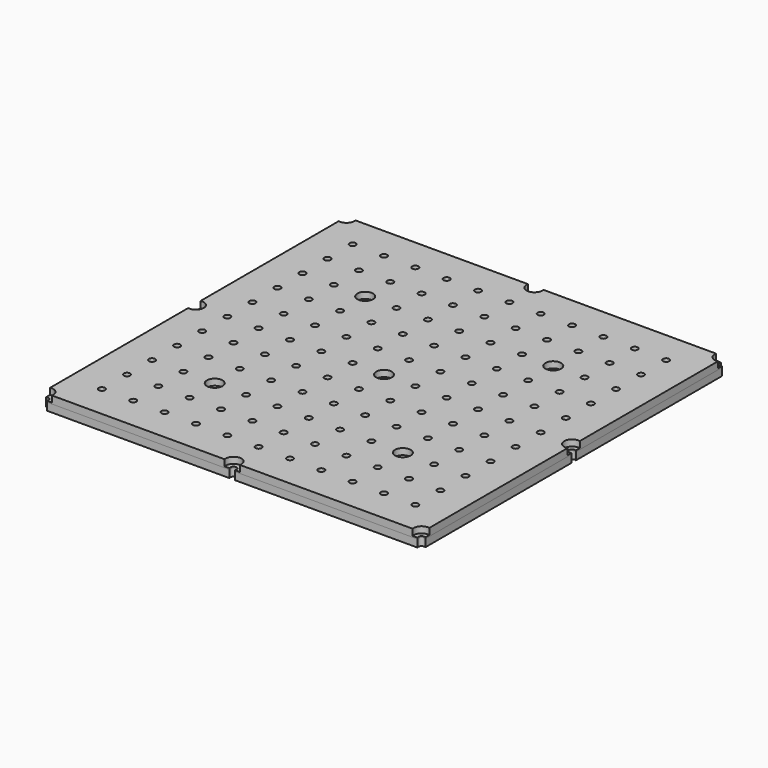
from build123d import *

# Parameters (mm, degrees)
F0_R     = 5
F1_DEPTH = 12
F2_R     = 5
F2_R_2   = 12.5
F3_DEPTH = 12
F4_R     = 5
F5_DEPTH = 2


with BuildPart() as f1:
    # F0 (on Top) → F1 (new body)
    with BuildSketch(Plane.XY):
        with BuildLine():
            ThreePointArc((302.5, 295.6698729811), (296.4644660941, 296.4644660941), (295.6698729811, 302.5))
            Line((295.6698729811, 302.5), (4.3301270189, 302.5))
            ThreePointArc((4.3301270189, 302.5), (0, 295), (-4.3301270189, 302.5))
            Line((-4.3301270189, 302.5), (-295.6698729811, 302.5))
            ThreePointArc((-295.6698729811, 302.5), (-296.4644660941, 296.4644660941), (-302.5, 295.6698729811))
            Line((-302.5, 295.6698729811), (-302.5, 4.3301270189))
            ThreePointArc((-302.5, 4.3301270189), (-295, 0), (-302.5, -4.3301270189))
            Line((-302.5, -4.3301270189), (-302.5, -295.6698729811))
            ThreePointArc((-302.5, -295.6698729811), (-296.4644660941, -296.4644660941), (-295.6698729811, -302.5))
            Line((-295.6698729811, -302.5), (-4.3301270189, -302.5))
            ThreePointArc((-4.3301270189, -302.5), (0, -295), (4.3301270189, -302.5))
            Line((4.3301270189, -302.5), (295.6698729811, -302.5))
            ThreePointArc((295.6698729811, -302.5), (296.4644660941, -296.4644660941), (302.5, -295.6698729811))
            Line((302.5, -295.6698729811), (302.5, -4.3301270189))
            ThreePointArc((302.5, -4.3301270189), (295, 0), (302.5, 4.3301270189))
            Line((302.5, 4.3301270189), (302.5, 295.6698729811))
        make_face()
        with Locations((-250, -250)):
            Circle(F0_R, mode=Mode.SUBTRACT)
        with Locations((-200, -250)):
            Circle(F0_R, mode=Mode.SUBTRACT)
        with Locations((-250, -200)):
            Circle(F0_R, mode=Mode.SUBTRACT)
        with Locations((-200, -200)):
            Circle(F0_R, mode=Mode.SUBTRACT)
        with Locations((-150, -250)):
            Circle(F0_R, mode=Mode.SUBTRACT)
        with Locations((-100, -250)):
            Circle(F0_R, mode=Mode.SUBTRACT)
        with Locations((-50, -250)):
            Circle(F0_R, mode=Mode.SUBTRACT)
        with Locations((-150, -200)):
            Circle(F0_R, mode=Mode.SUBTRACT)
        with Locations((-100, -200)):
            Circle(F0_R, mode=Mode.SUBTRACT)
        with Locations((-50, -200)):
            Circle(F0_R, mode=Mode.SUBTRACT)
        with Locations((-250, -150)):
            Circle(F0_R, mode=Mode.SUBTRACT)
        with Locations((-250, -100)):
            Circle(F0_R, mode=Mode.SUBTRACT)
        with Locations((-200, -150)):
            Circle(F0_R, mode=Mode.SUBTRACT)
        with Locations((-200, -100)):
            Circle(F0_R, mode=Mode.SUBTRACT)
        with Locations((-250, -50)):
            Circle(F0_R, mode=Mode.SUBTRACT)
        with Locations((-200, -50)):
            Circle(F0_R, mode=Mode.SUBTRACT)
        with Locations((-150, -150)):
            Circle(F0_R, mode=Mode.SUBTRACT)
        with Locations((-100, -150)):
            Circle(F0_R, mode=Mode.SUBTRACT)
        with Locations((-150, -100)):
            Circle(F0_R, mode=Mode.SUBTRACT)
        with Locations((-100, -100)):
            Circle(F0_R, mode=Mode.SUBTRACT)
        with Locations((-50, -150)):
            Circle(F0_R, mode=Mode.SUBTRACT)
        with Locations((-50, -100)):
            Circle(F0_R, mode=Mode.SUBTRACT)
        with Locations((-150, -50)):
            Circle(F0_R, mode=Mode.SUBTRACT)
        with Locations((-100, -50)):
            Circle(F0_R, mode=Mode.SUBTRACT)
        with Locations((-50, -50)):
            Circle(F0_R, mode=Mode.SUBTRACT)
        with Locations((0, -250)):
            Circle(F0_R, mode=Mode.SUBTRACT)
        with Locations((50, -250)):
            Circle(F0_R, mode=Mode.SUBTRACT)
        with Locations((100, -250)):
            Circle(F0_R, mode=Mode.SUBTRACT)
        with Locations((150, -250)):
            Circle(F0_R, mode=Mode.SUBTRACT)
        with Locations((0, -200)):
            Circle(F0_R, mode=Mode.SUBTRACT)
        with Locations((50, -200)):
            Circle(F0_R, mode=Mode.SUBTRACT)
        with Locations((100, -200)):
            Circle(F0_R, mode=Mode.SUBTRACT)
        with Locations((150, -200)):
            Circle(F0_R, mode=Mode.SUBTRACT)
        with Locations((200, -250)):
            Circle(F0_R, mode=Mode.SUBTRACT)
        with Locations((250, -250)):
            Circle(F0_R, mode=Mode.SUBTRACT)
        with Locations((200, -200)):
            Circle(F0_R, mode=Mode.SUBTRACT)
        with Locations((250, -200)):
            Circle(F0_R, mode=Mode.SUBTRACT)
        with Locations((0, -150)):
            Circle(F0_R, mode=Mode.SUBTRACT)
        with Locations((50, -150)):
            Circle(F0_R, mode=Mode.SUBTRACT)
        with Locations((0, -100)):
            Circle(F0_R, mode=Mode.SUBTRACT)
        with Locations((50, -100)):
            Circle(F0_R, mode=Mode.SUBTRACT)
        with Locations((100, -150)):
            Circle(F0_R, mode=Mode.SUBTRACT)
        with Locations((150, -150)):
            Circle(F0_R, mode=Mode.SUBTRACT)
        with Locations((100, -100)):
            Circle(F0_R, mode=Mode.SUBTRACT)
        with Locations((150, -100)):
            Circle(F0_R, mode=Mode.SUBTRACT)
        with Locations((0, -50)):
            Circle(F0_R, mode=Mode.SUBTRACT)
        with Locations((50, -50)):
            Circle(F0_R, mode=Mode.SUBTRACT)
        with Locations((100, -50)):
            Circle(F0_R, mode=Mode.SUBTRACT)
        with Locations((150, -50)):
            Circle(F0_R, mode=Mode.SUBTRACT)
        with Locations((200, -150)):
            Circle(F0_R, mode=Mode.SUBTRACT)
        with Locations((200, -100)):
            Circle(F0_R, mode=Mode.SUBTRACT)
        with Locations((250, -150)):
            Circle(F0_R, mode=Mode.SUBTRACT)
        with Locations((250, -100)):
            Circle(F0_R, mode=Mode.SUBTRACT)
        with Locations((200, -50)):
            Circle(F0_R, mode=Mode.SUBTRACT)
        with Locations((250, -50)):
            Circle(F0_R, mode=Mode.SUBTRACT)
        with Locations((-250, 0)):
            Circle(F0_R, mode=Mode.SUBTRACT)
        with Locations((-250, 50)):
            Circle(F0_R, mode=Mode.SUBTRACT)
        with Locations((-200, 0)):
            Circle(F0_R, mode=Mode.SUBTRACT)
        with Locations((-200, 50)):
            Circle(F0_R, mode=Mode.SUBTRACT)
        with Locations((-250, 100)):
            Circle(F0_R, mode=Mode.SUBTRACT)
        with Locations((-250, 150)):
            Circle(F0_R, mode=Mode.SUBTRACT)
        with Locations((-200, 100)):
            Circle(F0_R, mode=Mode.SUBTRACT)
        with Locations((-200, 150)):
            Circle(F0_R, mode=Mode.SUBTRACT)
        with Locations((-150, 0)):
            Circle(F0_R, mode=Mode.SUBTRACT)
        with Locations((-100, 0)):
            Circle(F0_R, mode=Mode.SUBTRACT)
        with Locations((-150, 50)):
            Circle(F0_R, mode=Mode.SUBTRACT)
        with Locations((-100, 50)):
            Circle(F0_R, mode=Mode.SUBTRACT)
        with Locations((-50, 0)):
            Circle(F0_R, mode=Mode.SUBTRACT)
        with Locations((-50, 50)):
            Circle(F0_R, mode=Mode.SUBTRACT)
        with Locations((-150, 100)):
            Circle(F0_R, mode=Mode.SUBTRACT)
        with Locations((-100, 100)):
            Circle(F0_R, mode=Mode.SUBTRACT)
        with Locations((-150, 150)):
            Circle(F0_R, mode=Mode.SUBTRACT)
        with Locations((-100, 150)):
            Circle(F0_R, mode=Mode.SUBTRACT)
        with Locations((-50, 100)):
            Circle(F0_R, mode=Mode.SUBTRACT)
        with Locations((-50, 150)):
            Circle(F0_R, mode=Mode.SUBTRACT)
        with Locations((-250, 200)):
            Circle(F0_R, mode=Mode.SUBTRACT)
        with Locations((-200, 200)):
            Circle(F0_R, mode=Mode.SUBTRACT)
        with Locations((-250, 250)):
            Circle(F0_R, mode=Mode.SUBTRACT)
        with Locations((-200, 250)):
            Circle(F0_R, mode=Mode.SUBTRACT)
        with Locations((-150, 200)):
            Circle(F0_R, mode=Mode.SUBTRACT)
        with Locations((-100, 200)):
            Circle(F0_R, mode=Mode.SUBTRACT)
        with Locations((-50, 200)):
            Circle(F0_R, mode=Mode.SUBTRACT)
        with Locations((-150, 250)):
            Circle(F0_R, mode=Mode.SUBTRACT)
        with Locations((-100, 250)):
            Circle(F0_R, mode=Mode.SUBTRACT)
        with Locations((-50, 250)):
            Circle(F0_R, mode=Mode.SUBTRACT)
        Circle(F0_R, mode=Mode.SUBTRACT)
        with Locations((50, 0)):
            Circle(F0_R, mode=Mode.SUBTRACT)
        with Locations((0, 50)):
            Circle(F0_R, mode=Mode.SUBTRACT)
        with Locations((50, 50)):
            Circle(F0_R, mode=Mode.SUBTRACT)
        with Locations((100, 0)):
            Circle(F0_R, mode=Mode.SUBTRACT)
        with Locations((150, 0)):
            Circle(F0_R, mode=Mode.SUBTRACT)
        with Locations((100, 50)):
            Circle(F0_R, mode=Mode.SUBTRACT)
        with Locations((150, 50)):
            Circle(F0_R, mode=Mode.SUBTRACT)
        with Locations((0, 100)):
            Circle(F0_R, mode=Mode.SUBTRACT)
        with Locations((50, 100)):
            Circle(F0_R, mode=Mode.SUBTRACT)
        with Locations((0, 150)):
            Circle(F0_R, mode=Mode.SUBTRACT)
        with Locations((50, 150)):
            Circle(F0_R, mode=Mode.SUBTRACT)
        with Locations((100, 100)):
            Circle(F0_R, mode=Mode.SUBTRACT)
        with Locations((150, 100)):
            Circle(F0_R, mode=Mode.SUBTRACT)
        with Locations((100, 150)):
            Circle(F0_R, mode=Mode.SUBTRACT)
        with Locations((150, 150)):
            Circle(F0_R, mode=Mode.SUBTRACT)
        with Locations((200, 0)):
            Circle(F0_R, mode=Mode.SUBTRACT)
        with Locations((200, 50)):
            Circle(F0_R, mode=Mode.SUBTRACT)
        with Locations((250, 0)):
            Circle(F0_R, mode=Mode.SUBTRACT)
        with Locations((250, 50)):
            Circle(F0_R, mode=Mode.SUBTRACT)
        with Locations((200, 100)):
            Circle(F0_R, mode=Mode.SUBTRACT)
        with Locations((200, 150)):
            Circle(F0_R, mode=Mode.SUBTRACT)
        with Locations((250, 100)):
            Circle(F0_R, mode=Mode.SUBTRACT)
        with Locations((250, 150)):
            Circle(F0_R, mode=Mode.SUBTRACT)
        with Locations((0, 200)):
            Circle(F0_R, mode=Mode.SUBTRACT)
        with Locations((50, 200)):
            Circle(F0_R, mode=Mode.SUBTRACT)
        with Locations((100, 200)):
            Circle(F0_R, mode=Mode.SUBTRACT)
        with Locations((150, 200)):
            Circle(F0_R, mode=Mode.SUBTRACT)
        with Locations((0, 250)):
            Circle(F0_R, mode=Mode.SUBTRACT)
        with Locations((50, 250)):
            Circle(F0_R, mode=Mode.SUBTRACT)
        with Locations((100, 250)):
            Circle(F0_R, mode=Mode.SUBTRACT)
        with Locations((150, 250)):
            Circle(F0_R, mode=Mode.SUBTRACT)
        with Locations((200, 200)):
            Circle(F0_R, mode=Mode.SUBTRACT)
        with Locations((250, 200)):
            Circle(F0_R, mode=Mode.SUBTRACT)
        with Locations((200, 250)):
            Circle(F0_R, mode=Mode.SUBTRACT)
        with Locations((250, 250)):
            Circle(F0_R, mode=Mode.SUBTRACT)
    extrude(amount=F1_DEPTH)


with BuildPart() as f3:
    # F2 (on face) → F3 (new body)
    with BuildSketch(Plane.XY.offset(12)):
        with BuildLine():
            ThreePointArc((-287.7525512861, 302.5), (-291.1611652352, 291.1611652352), (-302.5, 287.7525512861))
            Line((-302.5, 287.7525512861), (-302.5, 12.2474487139))
            ThreePointArc((-302.5, 12.2474487139), (-287.5, 0), (-302.5, -12.2474487139))
            Line((-302.5, -12.2474487139), (-302.5, -287.7525512861))
            ThreePointArc((-302.5, -287.7525512861), (-291.1611652352, -291.1611652352), (-287.7525512861, -302.5))
            Line((-287.7525512861, -302.5), (-12.2474487139, -302.5))
            ThreePointArc((-12.2474487139, -302.5), (0, -287.5), (12.2474487139, -302.5))
            Line((12.2474487139, -302.5), (287.7525512861, -302.5))
            ThreePointArc((287.7525512861, -302.5), (291.1611652352, -291.1611652352), (302.5, -287.7525512861))
            Line((302.5, -287.7525512861), (302.5, -12.2474487139))
            ThreePointArc((302.5, -12.2474487139), (287.5, 0), (302.5, 12.2474487139))
            Line((302.5, 12.2474487139), (302.5, 287.7525512861))
            ThreePointArc((302.5, 287.7525512861), (291.1611652352, 291.1611652352), (287.7525512861, 302.5))
            Line((287.7525512861, 302.5), (12.2474487139, 302.5))
            ThreePointArc((12.2474487139, 302.5), (0, 287.5), (-12.2474487139, 302.5))
            Line((-12.2474487139, 302.5), (-287.7525512861, 302.5))
        make_face()
        with Locations((-250, -250)):
            Circle(F2_R, mode=Mode.SUBTRACT)
        with Locations((-200, -250)):
            Circle(F2_R, mode=Mode.SUBTRACT)
        with Locations((-250, -200)):
            Circle(F2_R, mode=Mode.SUBTRACT)
        with Locations((-200, -200)):
            Circle(F2_R, mode=Mode.SUBTRACT)
        with Locations((-150, -250)):
            Circle(F2_R, mode=Mode.SUBTRACT)
        with Locations((-100, -250)):
            Circle(F2_R, mode=Mode.SUBTRACT)
        with Locations((-50, -250)):
            Circle(F2_R, mode=Mode.SUBTRACT)
        with Locations((-150, -200)):
            Circle(F2_R, mode=Mode.SUBTRACT)
        with Locations((-100, -200)):
            Circle(F2_R, mode=Mode.SUBTRACT)
        with Locations((-50, -200)):
            Circle(F2_R, mode=Mode.SUBTRACT)
        with Locations((-250, -150)):
            Circle(F2_R, mode=Mode.SUBTRACT)
        with Locations((-250, -100)):
            Circle(F2_R, mode=Mode.SUBTRACT)
        with Locations((-200, -150)):
            Circle(F2_R, mode=Mode.SUBTRACT)
        with Locations((-200, -100)):
            Circle(F2_R, mode=Mode.SUBTRACT)
        with Locations((-250, -50)):
            Circle(F2_R, mode=Mode.SUBTRACT)
        with Locations((-200, -50)):
            Circle(F2_R, mode=Mode.SUBTRACT)
        with Locations((-150, -150)):
            Circle(F2_R_2, mode=Mode.SUBTRACT)
        with Locations((-100, -150)):
            Circle(F2_R, mode=Mode.SUBTRACT)
        with Locations((-150, -100)):
            Circle(F2_R, mode=Mode.SUBTRACT)
        with Locations((-100, -100)):
            Circle(F2_R, mode=Mode.SUBTRACT)
        with Locations((-50, -150)):
            Circle(F2_R, mode=Mode.SUBTRACT)
        with Locations((-50, -100)):
            Circle(F2_R, mode=Mode.SUBTRACT)
        with Locations((-150, -50)):
            Circle(F2_R, mode=Mode.SUBTRACT)
        with Locations((-100, -50)):
            Circle(F2_R, mode=Mode.SUBTRACT)
        with Locations((-50, -50)):
            Circle(F2_R, mode=Mode.SUBTRACT)
        with Locations((0, -250)):
            Circle(F2_R, mode=Mode.SUBTRACT)
        with Locations((50, -250)):
            Circle(F2_R, mode=Mode.SUBTRACT)
        with Locations((100, -250)):
            Circle(F2_R, mode=Mode.SUBTRACT)
        with Locations((150, -250)):
            Circle(F2_R, mode=Mode.SUBTRACT)
        with Locations((0, -200)):
            Circle(F2_R, mode=Mode.SUBTRACT)
        with Locations((50, -200)):
            Circle(F2_R, mode=Mode.SUBTRACT)
        with Locations((100, -200)):
            Circle(F2_R, mode=Mode.SUBTRACT)
        with Locations((150, -200)):
            Circle(F2_R, mode=Mode.SUBTRACT)
        with Locations((200, -250)):
            Circle(F2_R, mode=Mode.SUBTRACT)
        with Locations((250, -250)):
            Circle(F2_R, mode=Mode.SUBTRACT)
        with Locations((200, -200)):
            Circle(F2_R, mode=Mode.SUBTRACT)
        with Locations((250, -200)):
            Circle(F2_R, mode=Mode.SUBTRACT)
        with Locations((0, -150)):
            Circle(F2_R, mode=Mode.SUBTRACT)
        with Locations((50, -150)):
            Circle(F2_R, mode=Mode.SUBTRACT)
        with Locations((0, -100)):
            Circle(F2_R, mode=Mode.SUBTRACT)
        with Locations((50, -100)):
            Circle(F2_R, mode=Mode.SUBTRACT)
        with Locations((100, -150)):
            Circle(F2_R, mode=Mode.SUBTRACT)
        with Locations((150, -150)):
            Circle(F2_R_2, mode=Mode.SUBTRACT)
        with Locations((100, -100)):
            Circle(F2_R, mode=Mode.SUBTRACT)
        with Locations((150, -100)):
            Circle(F2_R, mode=Mode.SUBTRACT)
        with Locations((0, -50)):
            Circle(F2_R, mode=Mode.SUBTRACT)
        with Locations((50, -50)):
            Circle(F2_R, mode=Mode.SUBTRACT)
        with Locations((100, -50)):
            Circle(F2_R, mode=Mode.SUBTRACT)
        with Locations((150, -50)):
            Circle(F2_R, mode=Mode.SUBTRACT)
        with Locations((200, -150)):
            Circle(F2_R, mode=Mode.SUBTRACT)
        with Locations((200, -100)):
            Circle(F2_R, mode=Mode.SUBTRACT)
        with Locations((250, -150)):
            Circle(F2_R, mode=Mode.SUBTRACT)
        with Locations((250, -100)):
            Circle(F2_R, mode=Mode.SUBTRACT)
        with Locations((200, -50)):
            Circle(F2_R, mode=Mode.SUBTRACT)
        with Locations((250, -50)):
            Circle(F2_R, mode=Mode.SUBTRACT)
        with Locations((-250, 0)):
            Circle(F2_R, mode=Mode.SUBTRACT)
        with Locations((-250, 50)):
            Circle(F2_R, mode=Mode.SUBTRACT)
        with Locations((-200, 0)):
            Circle(F2_R, mode=Mode.SUBTRACT)
        with Locations((-200, 50)):
            Circle(F2_R, mode=Mode.SUBTRACT)
        with Locations((-250, 100)):
            Circle(F2_R, mode=Mode.SUBTRACT)
        with Locations((-250, 150)):
            Circle(F2_R, mode=Mode.SUBTRACT)
        with Locations((-200, 100)):
            Circle(F2_R, mode=Mode.SUBTRACT)
        with Locations((-200, 150)):
            Circle(F2_R, mode=Mode.SUBTRACT)
        with Locations((-150, 0)):
            Circle(F2_R, mode=Mode.SUBTRACT)
        with Locations((-100, 0)):
            Circle(F2_R, mode=Mode.SUBTRACT)
        with Locations((-150, 50)):
            Circle(F2_R, mode=Mode.SUBTRACT)
        with Locations((-100, 50)):
            Circle(F2_R, mode=Mode.SUBTRACT)
        with Locations((-50, 0)):
            Circle(F2_R, mode=Mode.SUBTRACT)
        with Locations((-50, 50)):
            Circle(F2_R, mode=Mode.SUBTRACT)
        with Locations((-150, 100)):
            Circle(F2_R, mode=Mode.SUBTRACT)
        with Locations((-100, 100)):
            Circle(F2_R, mode=Mode.SUBTRACT)
        with Locations((-150, 150)):
            Circle(F2_R_2, mode=Mode.SUBTRACT)
        with Locations((-100, 150)):
            Circle(F2_R, mode=Mode.SUBTRACT)
        with Locations((-50, 100)):
            Circle(F2_R, mode=Mode.SUBTRACT)
        with Locations((-50, 150)):
            Circle(F2_R, mode=Mode.SUBTRACT)
        with Locations((-250, 200)):
            Circle(F2_R, mode=Mode.SUBTRACT)
        with Locations((-200, 200)):
            Circle(F2_R, mode=Mode.SUBTRACT)
        with Locations((-250, 250)):
            Circle(F2_R, mode=Mode.SUBTRACT)
        with Locations((-200, 250)):
            Circle(F2_R, mode=Mode.SUBTRACT)
        with Locations((-150, 200)):
            Circle(F2_R, mode=Mode.SUBTRACT)
        with Locations((-100, 200)):
            Circle(F2_R, mode=Mode.SUBTRACT)
        with Locations((-50, 200)):
            Circle(F2_R, mode=Mode.SUBTRACT)
        with Locations((-150, 250)):
            Circle(F2_R, mode=Mode.SUBTRACT)
        with Locations((-100, 250)):
            Circle(F2_R, mode=Mode.SUBTRACT)
        with Locations((-50, 250)):
            Circle(F2_R, mode=Mode.SUBTRACT)
        Circle(F2_R_2, mode=Mode.SUBTRACT)
        with Locations((50, 0)):
            Circle(F2_R, mode=Mode.SUBTRACT)
        with Locations((0, 50)):
            Circle(F2_R, mode=Mode.SUBTRACT)
        with Locations((50, 50)):
            Circle(F2_R, mode=Mode.SUBTRACT)
        with Locations((100, 0)):
            Circle(F2_R, mode=Mode.SUBTRACT)
        with Locations((150, 0)):
            Circle(F2_R, mode=Mode.SUBTRACT)
        with Locations((100, 50)):
            Circle(F2_R, mode=Mode.SUBTRACT)
        with Locations((150, 50)):
            Circle(F2_R, mode=Mode.SUBTRACT)
        with Locations((0, 100)):
            Circle(F2_R, mode=Mode.SUBTRACT)
        with Locations((50, 100)):
            Circle(F2_R, mode=Mode.SUBTRACT)
        with Locations((0, 150)):
            Circle(F2_R, mode=Mode.SUBTRACT)
        with Locations((50, 150)):
            Circle(F2_R, mode=Mode.SUBTRACT)
        with Locations((100, 100)):
            Circle(F2_R, mode=Mode.SUBTRACT)
        with Locations((150, 100)):
            Circle(F2_R, mode=Mode.SUBTRACT)
        with Locations((100, 150)):
            Circle(F2_R, mode=Mode.SUBTRACT)
        with Locations((150, 150)):
            Circle(F2_R_2, mode=Mode.SUBTRACT)
        with Locations((200, 0)):
            Circle(F2_R, mode=Mode.SUBTRACT)
        with Locations((200, 50)):
            Circle(F2_R, mode=Mode.SUBTRACT)
        with Locations((250, 0)):
            Circle(F2_R, mode=Mode.SUBTRACT)
        with Locations((250, 50)):
            Circle(F2_R, mode=Mode.SUBTRACT)
        with Locations((200, 100)):
            Circle(F2_R, mode=Mode.SUBTRACT)
        with Locations((200, 150)):
            Circle(F2_R, mode=Mode.SUBTRACT)
        with Locations((250, 100)):
            Circle(F2_R, mode=Mode.SUBTRACT)
        with Locations((250, 150)):
            Circle(F2_R, mode=Mode.SUBTRACT)
        with Locations((0, 200)):
            Circle(F2_R, mode=Mode.SUBTRACT)
        with Locations((50, 200)):
            Circle(F2_R, mode=Mode.SUBTRACT)
        with Locations((100, 200)):
            Circle(F2_R, mode=Mode.SUBTRACT)
        with Locations((150, 200)):
            Circle(F2_R, mode=Mode.SUBTRACT)
        with Locations((0, 250)):
            Circle(F2_R, mode=Mode.SUBTRACT)
        with Locations((50, 250)):
            Circle(F2_R, mode=Mode.SUBTRACT)
        with Locations((100, 250)):
            Circle(F2_R, mode=Mode.SUBTRACT)
        with Locations((150, 250)):
            Circle(F2_R, mode=Mode.SUBTRACT)
        with Locations((200, 200)):
            Circle(F2_R, mode=Mode.SUBTRACT)
        with Locations((250, 200)):
            Circle(F2_R, mode=Mode.SUBTRACT)
        with Locations((200, 250)):
            Circle(F2_R, mode=Mode.SUBTRACT)
        with Locations((250, 250)):
            Circle(F2_R, mode=Mode.SUBTRACT)
    extrude(amount=F3_DEPTH)

    # F4 (on face) → F5 (join)
    with BuildSketch(Plane.XY.offset(12)):
        with BuildLine():
            ThreePointArc((302.5, 295.6698729811), (296.4644660941, 296.4644660941), (295.6698729811, 302.5))
            Line((295.6698729811, 302.5), (4.3301270189, 302.5))
            ThreePointArc((4.3301270189, 302.5), (0, 295), (-4.3301270189, 302.5))
            Line((-4.3301270189, 302.5), (-295.6698729811, 302.5))
            ThreePointArc((-295.6698729811, 302.5), (-296.4644660941, 296.4644660941), (-302.5, 295.6698729811))
            Line((-302.5, 295.6698729811), (-302.5, 4.3301270189))
            ThreePointArc((-302.5, 4.3301270189), (-295, 0), (-302.5, -4.3301270189))
            Line((-302.5, -4.3301270189), (-302.5, -295.6698729811))
            ThreePointArc((-302.5, -295.6698729811), (-296.4644660941, -296.4644660941), (-295.6698729811, -302.5))
            Line((-295.6698729811, -302.5), (-4.3301270189, -302.5))
            ThreePointArc((-4.3301270189, -302.5), (0, -295), (4.3301270189, -302.5))
            Line((4.3301270189, -302.5), (295.6698729811, -302.5))
            ThreePointArc((295.6698729811, -302.5), (296.4644660941, -296.4644660941), (302.5, -295.6698729811))
            Line((302.5, -295.6698729811), (302.5, -4.3301270189))
            ThreePointArc((302.5, -4.3301270189), (295, 0), (302.5, 4.3301270189))
            Line((302.5, 4.3301270189), (302.5, 295.6698729811))
        make_face()
        with Locations((-150, -150)):
            Circle(F4_R, mode=Mode.SUBTRACT)
        with Locations((150, -150)):
            Circle(F4_R, mode=Mode.SUBTRACT)
        with Locations((-150, 150)):
            Circle(F4_R, mode=Mode.SUBTRACT)
        Circle(F4_R, mode=Mode.SUBTRACT)
        with Locations((150, 150)):
            Circle(F4_R, mode=Mode.SUBTRACT)
    extrude(amount=F5_DEPTH)


solid = Compound([f1.part, f3.part])
